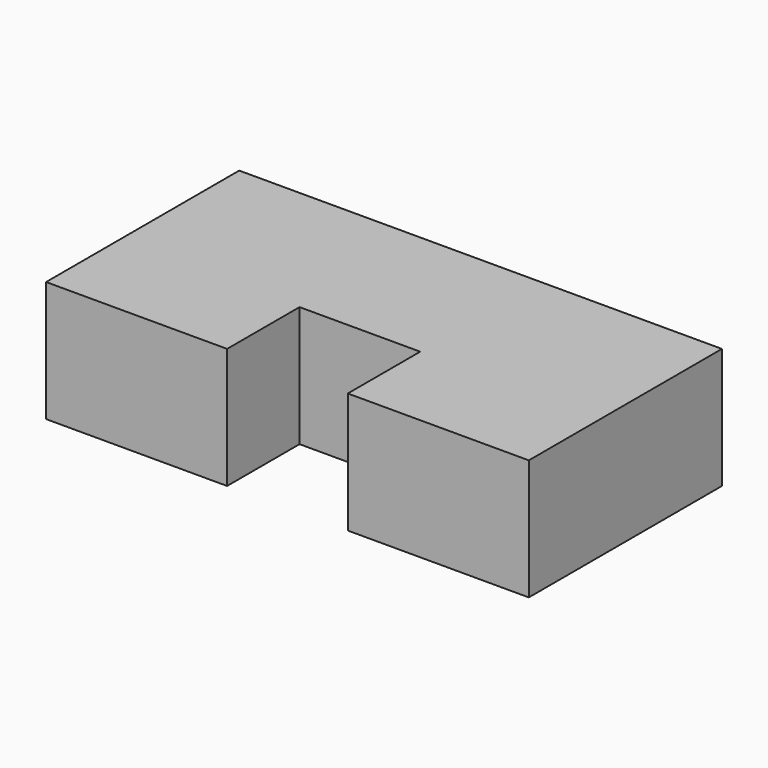
from build123d import *

# Parameters (mm, degrees)
F1_DEPTH = 25.4


# Not quite as in the source:
# - the program builds the solid bodies; features that only make, move or delete a surface that nothing else refers to are left out


with BuildPart() as f1:
    # F0 (on Top) → F1 (new body)
    with BuildSketch(Plane.XY):
        Polygon((0, 50.8), (0, 0), (38.1, 0), (38.1, 19.05), (63.5, 19.05), (63.5, 0), (101.6, 0), (101.6, 50.8), align=None)
    extrude(amount=F1_DEPTH)


solid = f1.part
